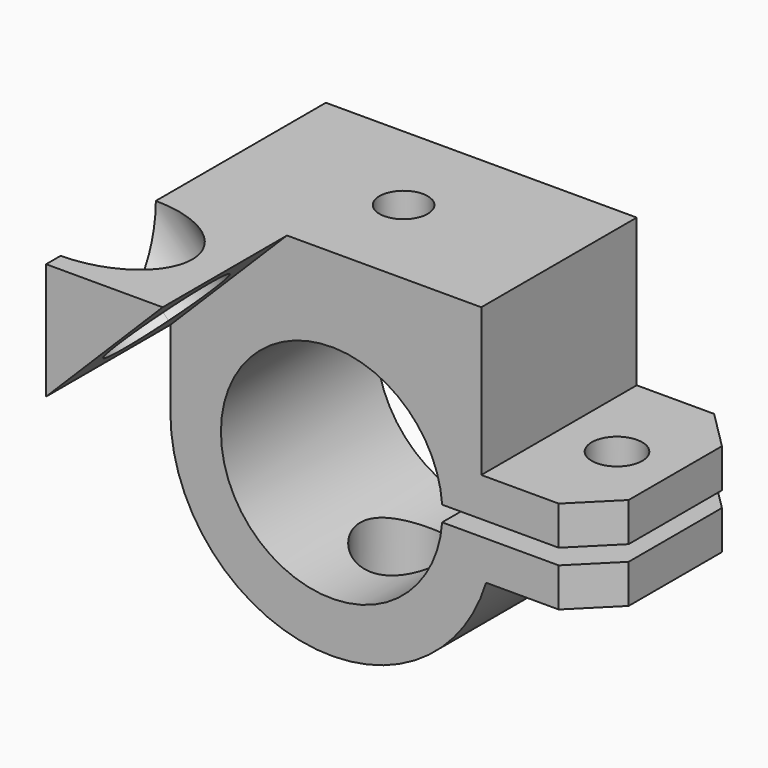
from build123d import *

# Parameters (mm, degrees)
F1_DEPTH       = 25
F4_D           = 6.2
F4_DEPTH       = 15
F4_START       = 14.2500001
F4_CBORE_D     = 11.13
F4_CBORE_DEPTH = 6.2
F4_TIP         = 1.862667919
F6_D           = 6.5
F6_DEPTH       = 15
F6_TIP         = 1.9527970118
F7_D           = 11.13
F7_DEPTH       = 15
F7_START       = 14.2500001
F7_TIP         = 3.3437893449
F8_SIZE        = 5
F10_DEPTH      = 20
F12_DEPTH      = 25


with BuildPart() as f1:
    # F0 (on Front) → F1 (new body)
    with BuildSketch(Plane.XZ):
        with BuildLine():
            ThreePointArc((14.2148689744, -1.0000000203), (-14.25, 2.03e-08), (14.2148689773, 0.9999999797))
            Line((14.2148689773, 0.9999999797), (34.2148689773, 0.9999999512))
            Line((34.2148689773, 0.9999999512), (34.2148682392, 6.0000000034))
            Line((34.2148682392, 6.0000000034), (19.2499992919, 6.0000000247))
            Line((19.2499992919, 6.0000000247), (19.2499992919, 25))
            Line((19.2499992919, 25), (-20.7500007081, 25))
            Line((-20.7500007081, 25), (-20.7500007081, 0))
            ThreePointArc((-20.7500007081, 0), (-3.0325612089, -20.5272039474), (19.8635980891, -6.0000000283))
            Line((19.8635980891, -6.0000000283), (34.2148682221, -6.0000000488))
            Line((34.2148682221, -6.0000000488), (34.2148689744, -1.0000000488))
            Line((34.2148689744, -1.0000000488), (14.2148689744, -1.0000000203))
        make_face()
    extrude(amount=F1_DEPTH)

    # F4
    # its depths count from where the whole tool has entered the part; down to there all is cleared
    with Locations(Plane(origin=(0, 0, 0), x_dir=(1, 0, 0), z_dir=(0, 0, -1)).offset(-F4_START)):
        with Locations((-0.7500007081, 12.5)):
            CounterBoreHole(F4_D / 2, F4_CBORE_D / 2, F4_CBORE_DEPTH, depth=F4_DEPTH)
            with Locations((0, 0, -(F4_DEPTH + F4_TIP / 2))):  # 118° drill point
                Cone(0, F4_D / 2, F4_TIP, mode=Mode.SUBTRACT)

    # F6
    with Locations(Plane(origin=(8.6e-09, 0, 6.0000000522), x_dir=(1, 0, -1.4e-09), z_dir=(1.4e-09, 0, 1))):
        with Locations((26.7148682306, -12.5)):
            Hole(F6_D / 2, depth=F6_DEPTH)
            with Locations((0, 0, -(F6_DEPTH + F6_TIP / 2))):  # 118° drill point
                Cone(0, F6_D / 2, F6_TIP, mode=Mode.SUBTRACT)

    # F7
    # its depths count from where the whole tool has entered the part; down to there all is cleared
    with Locations(Plane.XY.offset(-F7_START)):
        with Locations((-0.7500007081, -12.5)):
            Hole(F7_D / 2, depth=F7_DEPTH)
            with Locations((0, 0, -(F7_DEPTH + F7_TIP / 2))):  # 118° drill point
                Cone(0, F7_D / 2, F7_TIP, mode=Mode.SUBTRACT)

    # F8
    f8_edges = [f1.edges().sort_by_distance(p)[0] for p in [
        (34.214869, -25, 3.5),
        (34.214869, -25, -3.5),
        (34.214869, 0, -3.5),
        (34.214869, 0, 3.5),
    ]]
    chamfer(f8_edges, length=F8_SIZE)

    # F9 (on face) → F10 (join)
    with BuildSketch(Plane.XZ.offset(25)):
        Polygon((-5.7500007081, 25), (-20.7500007081, 25), (-20.7500007081, 10), align=None)
    extrude(amount=F10_DEPTH)

    # F11 (on face) → F12 (cut)
    with BuildSketch(Plane(origin=(-15.375000354, 0, 15.375000354), x_dir=(0.7071067812, 0, 0.7071067812), z_dir=(0.7071067812, 0, -0.7071067812))):
        with BuildLine():
            Line((3.0052033194, 35), (8.5698333836, 40.2463835376))
            ThreePointArc((8.5698333836, 40.2463835376), (3.0052033194, 42.6478525074), (-2.5594267448, 40.2463835376))
            Line((-2.5594267448, 40.2463835376), (3.0052033194, 35))
        make_face()
        with BuildLine():
            Line((-2.5594267448, 29.7536164624), (3.0052033194, 35))
            Line((3.0052033194, 35), (-2.5594267448, 40.2463835376))
            ThreePointArc((-2.5594267448, 40.2463835376), (-4.642649188, 35), (-2.5594267448, 29.7536164624))
        make_face()
        with BuildLine():
            ThreePointArc((10.6530558268, 35), (10.1131959321, 37.8224260828), (8.5698333836, 40.2463835376))
            Line((8.5698333836, 40.2463835376), (3.0052033194, 35))
            Line((3.0052033194, 35), (8.5698333836, 29.7536164624))
            ThreePointArc((8.5698333836, 29.7536164624), (10.1131959321, 32.1775739172), (10.6530558268, 35))
        make_face()
        with BuildLine():
            Line((8.5698333836, 29.7536164624), (3.0052033194, 35))
            Line((3.0052033194, 35), (-2.5594267448, 29.7536164624))
            ThreePointArc((-2.5594267448, 29.7536164624), (3.0052033194, 27.3521474926), (8.5698333836, 29.7536164624))
        make_face()
    extrude(amount=-F12_DEPTH, mode=Mode.SUBTRACT)


solid = f1.part
